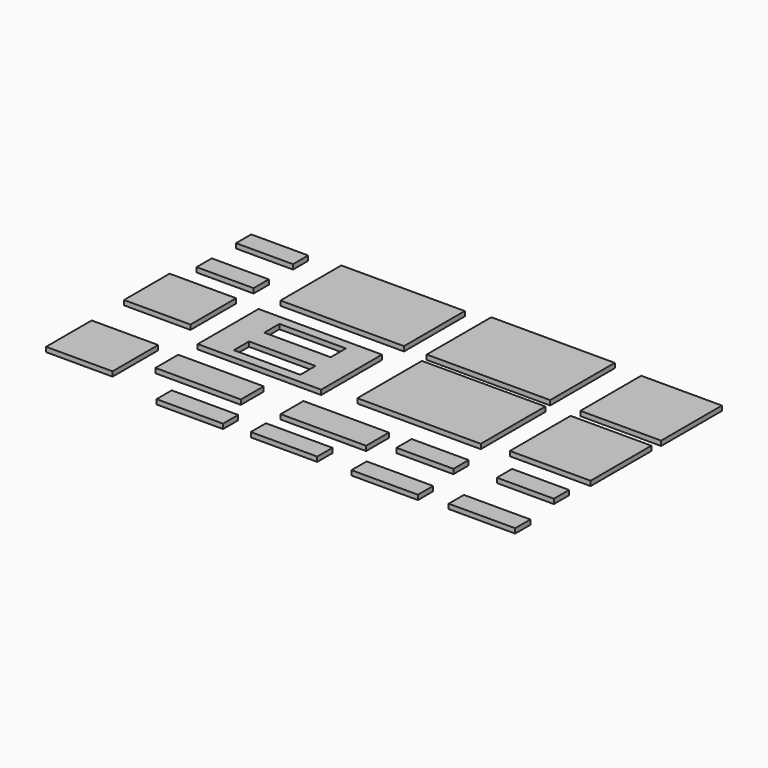
from build123d import *

# Parameters (mm, degrees)
F1_W     = 76.2
F1_H     = 25.4
F2_DEPTH = 6.35
F1_W_2   = 88.9
F1_H_2   = 76.2
F1_W_3   = 165.1
F1_H_3   = 101.6
F1_W_4   = 114.3
F1_H_4   = 38.1
F1_W_5   = 107.95
F1_H_5   = 107.95


# Not quite as in the source:
# - a variable given as a bare number and used for a length is read in inches; the dataset says mm whatever the document's units were


with BuildPart() as f2:
    # F1 (on Top) → F2 (new body)
    with BuildSketch(Plane.XY):
        with Locations((-423.1286319411, 99.3716068767)):
            Rectangle(F1_W, F1_H)
    extrude(amount=F2_DEPTH)


with BuildPart() as f2b:
    # F1 (on Top) → F2, piece 2 (new body)
    with BuildSketch(Plane.XY):
        with Locations((-421.4286606973, 31.3716022751)):
            Rectangle(F1_W, F1_H)
    extrude(amount=F2_DEPTH)


with BuildPart() as f2c:
    # F1 (on Top) → F2, piece 3 (new body)
    with BuildSketch(Plane.XY):
        with Locations((-427.8286524599, -48.6284039599)):
            Rectangle(F1_W_2, F1_H_2)
    extrude(amount=F2_DEPTH)


with BuildPart() as f2d:
    # F1 (on Top) → F2, piece 4 (new body)
    with BuildSketch(Plane.XY):
        with Locations((-425.2786477248, -182.0783964606)):
            Rectangle(F1_W_2, F1_H_2)
    extrude(amount=F2_DEPTH)


with BuildPart() as f2e:
    # F1 (on Top) → F2, piece 5 (new body)
    with BuildSketch(Plane.XY):
        with Locations((-261.3786375164, 65.2216013642)):
            Rectangle(F1_W_3, F1_H_3)
    extrude(amount=F2_DEPTH)


with BuildPart() as f2f:
    # F1 (on Top) → F2, piece 6 (new body)
    with BuildSketch(Plane.XY):
        with Locations((-267.328648565, -65.6784033552)):
            Rectangle(F1_W_3, F1_H_3)
        with Locations((-267.328648565, -91.0784033552)):
            Rectangle(F1_W_2, F1_H, mode=Mode.SUBTRACT)
        with Locations((-267.328648565, -40.2784033552)):
            Rectangle(F1_W_2, F1_H, mode=Mode.SUBTRACT)
    extrude(amount=F2_DEPTH)


with BuildPart() as f2g:
    # F1 (on Top) → F2, piece 7 (new body)
    with BuildSketch(Plane.XY):
        with Locations((-293.5786501434, -167.1283971517)):
            Rectangle(F1_W_4, F1_H_4)
    extrude(amount=F2_DEPTH)


with BuildPart() as f2h:
    # F1 (on Top) → F2, piece 8 (new body)
    with BuildSketch(Plane.XY):
        with Locations((-261.2286622286, -227.8784024286)):
            Rectangle(F1_W_2, F1_H)
    extrude(amount=F2_DEPTH)


with BuildPart() as f2i:
    # F1 (on Top) → F2, piece 9 (new body)
    with BuildSketch(Plane.XY):
        with Locations((-126.1286423772, -167.1283971517)):
            Rectangle(F1_W_4, F1_H_4)
    extrude(amount=F2_DEPTH)


with BuildPart() as f2j:
    # F1 (on Top) → F2, piece 10 (new body)
    with BuildSketch(Plane.XY):
        with Locations((-137.9786567553, -224.4784120716)):
            Rectangle(F1_W_2, F1_H)
    extrude(amount=F2_DEPTH)


with BuildPart() as f2k:
    # F1 (on Top) → F2, piece 11 (new body)
    with BuildSketch(Plane.XY):
        with Locations((-3.2286500492, -157.3283990755)):
            Rectangle(F1_W, F1_H)
    extrude(amount=F2_DEPTH)


with BuildPart() as f2l:
    # F1 (on Top) → F2, piece 12 (new body)
    with BuildSketch(Plane.XY):
        with Locations((-1.9786435629, -226.1784152283)):
            Rectangle(F1_W_2, F1_H)
    extrude(amount=F2_DEPTH)


with BuildPart() as f2m:
    # F1 (on Top) → F2, piece 13 (new body)
    with BuildSketch(Plane.XY):
        with Locations((124.6713682238, -221.9284073365)):
            Rectangle(F1_W_2, F1_H)
    extrude(amount=F2_DEPTH)


with BuildPart() as f2n:
    # F1 (on Top) → F2, piece 14 (new body)
    with BuildSketch(Plane.XY):
        with Locations((120.8713649807, -144.5784073129)):
            Rectangle(F1_W, F1_H)
    extrude(amount=F2_DEPTH)


with BuildPart() as f2o:
    # F1 (on Top) → F2, piece 15 (new body)
    with BuildSketch(Plane.XY):
        with Locations((109.5463703205, -50.8)):
            Rectangle(F1_W_5, F1_H_3)
    extrude(amount=F2_DEPTH)


with BuildPart() as f2p:
    # F1 (on Top) → F2, piece 16 (new body)
    with BuildSketch(Plane.XY):
        with Locations((110.396343975, 66.0715989535)):
            Rectangle(F1_W_5, F1_H_3)
    extrude(amount=F2_DEPTH)


with BuildPart() as f2q:
    # F1 (on Top) → F2, piece 17 (new body)
    with BuildSketch(Plane.XY):
        with Locations((-65.8786574463, 68.3966013642)):
            Rectangle(F1_W_3, F1_H_5)
    extrude(amount=F2_DEPTH)


with BuildPart() as f2r:
    # F1 (on Top) → F2, piece 18 (new body)
    with BuildSketch(Plane.XY):
        with Locations((-60.7786479761, -53.975)):
            Rectangle(F1_W_3, F1_H_5)
    extrude(amount=F2_DEPTH)


solid = Compound([f2.part, f2b.part, f2c.part, f2d.part, f2e.part, f2f.part, f2g.part, f2h.part, f2i.part, f2j.part, f2k.part, f2l.part, f2m.part, f2n.part, f2o.part, f2p.part, f2q.part, f2r.part])
